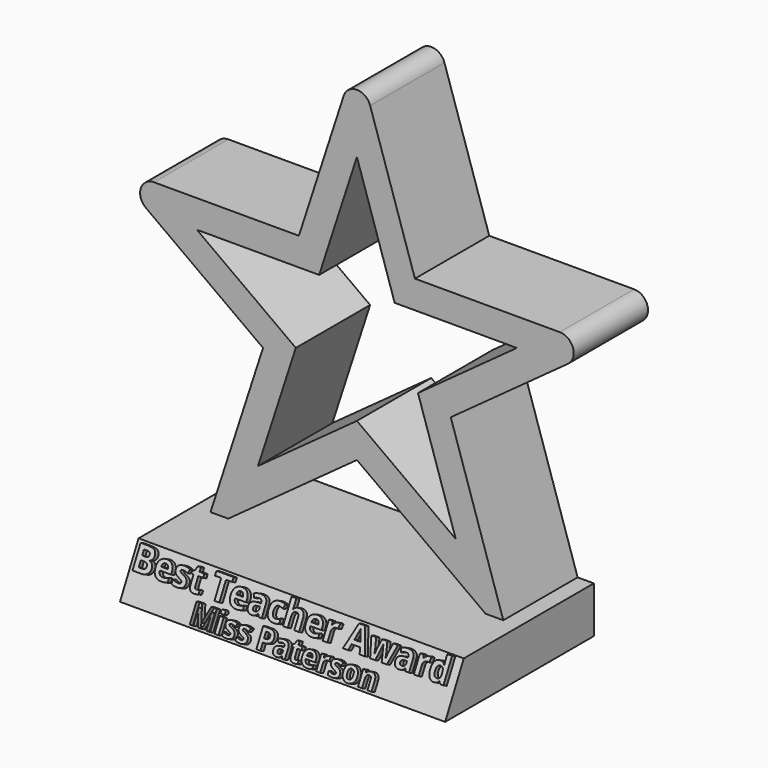
from build123d import *

# Parameters (mm, degrees)
F1_DEPTH       = 20
F2_R           = 3
F4_DEPTH       = 35
F5_DEPTH       = 35
F6_TEXT_SIZE   = 6.8495522294
F6_TEXT_SIZE_2 = 5.7339963267
F7_DEPTH       = 1


# Not quite as in the source:
# - Text() gives the source's letters only with a copy of the font that has no kerning and outlines rounded to 1/6400 em; it was checked with that copy


with BuildPart() as f1:
    # F0 (on Front) → F1 (new body)
    with BuildSketch(Plane.XZ):
        Polygon((-12.4881548142, 67.1884705063), (-52.9006727063, 67.1884705063), (-20.2062589461, 43.4345884812), (-31.5140738727, 8.63271264), (-27.6944137602, 8.63271264), (0, 28.753882025), (27.6944137602, 8.63271264), (31.5140738727, 8.63271264), (20.2062589461, 43.4345884812), (52.9006727063, 67.1884705063), (12.4881548142, 67.1884705063), (0, 105.6230589875), align=None)
        Polygon((-13.1528359186, 45.7263845487), (-34.4345714833, 61.1884705063), (-8.1288996461, 61.1884705063), (0, 86.2066511225), (8.1288996461, 61.1884705063), (34.4345714833, 61.1884705063), (13.1528359186, 45.7263845487), (21.2817355647, 20.7082039325), (0, 36.17028989), (-21.2817355647, 20.7082039325), align=None, mode=Mode.SUBTRACT)
    extrude(amount=F1_DEPTH)

    # F2
    f2_edges = [f1.edges().sort_by_distance(p)[0] for p in [
        (0, -10, 105.623059),
        (-52.900673, -10, 67.188471),
        (52.900673, -10, 67.188471),
    ]]
    fillet(f2_edges, radius=F2_R)

    # F3 (on Right) → F4 (join)
    with BuildSketch(Plane.YZ):
        Polygon((0, 8.63271264), (-20, 8.63271264), (-35, 8.63271264), (-40, -1.36728736), (0, -1.36728736), align=None)
    extrude(amount=F4_DEPTH)

    # F5 (add): a face of the model
    f5_faces = [f1.faces().sort_by_distance(p)[0] for p in [
        (0, -18.7777777778, 3.5216015289),
    ]]
    extrude(f5_faces, amount=F5_DEPTH)

    # F6 (on face) → F7 (join)
    with BuildSketch(Plane(origin=(0, -31.453085056, 15.726542528), x_dir=(1, 0, 0), z_dir=(0, -0.894427191, 0.4472135955))):
        with Locations((-34.2988449916, -13.2849395909)):
            Text('Best Teacher Award', F6_TEXT_SIZE, font='Open Sans', font_style=FontStyle.BOLD, text_align=(TextAlign.LEFT, TextAlign.BOTTOM))
        with Locations((-20, -18.5157900314)):
            Text('Miss Paterson', F6_TEXT_SIZE_2, font='Open Sans', font_style=FontStyle.BOLD, text_align=(TextAlign.LEFT, TextAlign.BOTTOM))
    extrude(amount=F7_DEPTH)


solid = f1.part
